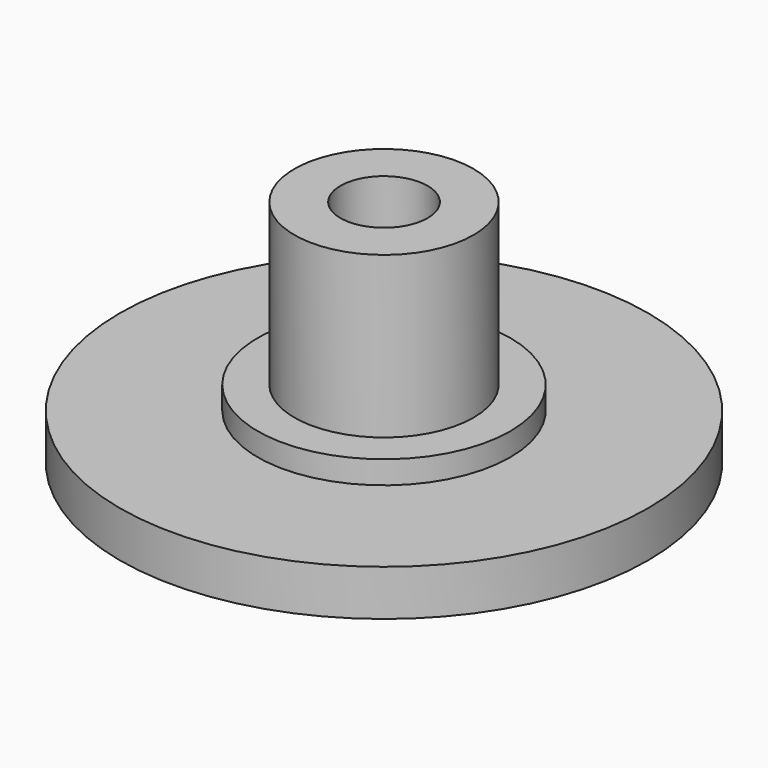
from build123d import *

# Parameters (mm, degrees)
F0_R         = 11.5
F1_DEPTH     = 2
F2_R         = 5.5
F3_DEPTH     = 1
F4_R         = 3.9
F5_DEPTH     = 7
F6_R         = 1.9
F7_DEPTH     = 7
F8_TEXT_SIZE = 20.557991229
F9_DEPTH     = 1


# Not quite as in the source:
# - Text() gives the source's letters only with a copy of the font that has no kerning and outlines rounded to 1/6400 em; it was checked with that copy


with BuildPart() as f1:
    # F0 (on Top) → F1 (new body)
    with BuildSketch(Plane.XY):
        Circle(F0_R)
    extrude(amount=F1_DEPTH)

    # F2 (on face) → F3 (join)
    with BuildSketch(Plane.XY.offset(2)):
        Circle(F2_R)
    extrude(amount=F3_DEPTH)

    # F4 (on face) → F5 (join)
    with BuildSketch(Plane.XY.offset(3)):
        Circle(F4_R)
    extrude(amount=F5_DEPTH)

    # F6 (on face) → F7 (cut)
    with BuildSketch(Plane.XY.offset(10)):
        Circle(F6_R)
    extrude(amount=-F7_DEPTH, mode=Mode.SUBTRACT)

    # F8 (on face) → F9 (cut)
    with BuildSketch(Plane(origin=(0, 0, 0), x_dir=(1, 0, 0), z_dir=(0, 0, -1))):
        with Locations((-5.2809744666, -7.4764034944)):
            Text('P', F8_TEXT_SIZE, font='Open Sans', text_align=(TextAlign.LEFT, TextAlign.BOTTOM))
    extrude(amount=-F9_DEPTH, mode=Mode.SUBTRACT)


solid = f1.part
